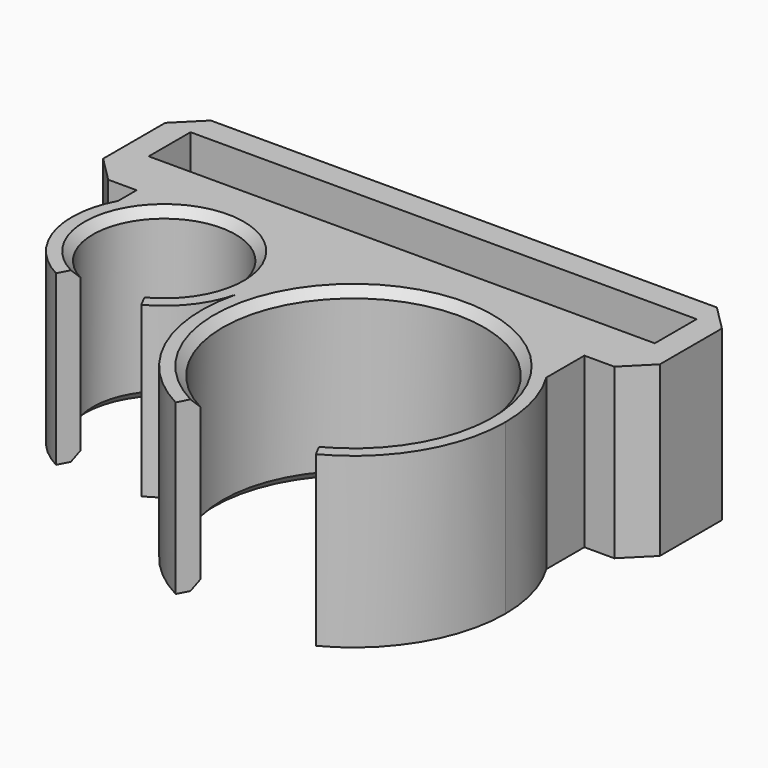
from build123d import *

# Parameters (mm, degrees)
F0_W          = 60
F0_H          = 6.2
F0_R          = 8.45
F0_R_2        = 15.5
F1_DEPTH      = 20
F2_SIZE       = 1
F4_W          = 48.1594242923
F4_H          = 40.4543727636
F5_ANGLE_BACK = 27.5
F5_ANGLE      = 55
F7_W          = 69.6530229799
F7_H          = 48.1908544898
F8_ANGLE_BACK = 27.5
F8_ANGLE      = 55
F9_SIZE       = 3
F10_SIZE      = 3
F11_SIZE      = 3
F12_SIZE      = 1
F13_TEXT_SIZE = 11.0604027416
F14_DEPTH     = 4
F15_DEPTH     = 0.8157047022


# Not quite as in the source:
# - Text() gives the source's letters only with a copy of the font that has no kerning and outlines rounded to 1/6400 em; it was checked with that copy


with BuildPart() as f1:
    # F0 (on Top) → F1 (new body)
    with BuildSketch(Plane.XY):
        Polygon((-2.1916090953, 0.4419453137), (-2.1916090953, -11.7580546863), (13.8083908874, -11.7580546863), (41.886852401, -11.7580546863), (63.8083909047, -11.7580546863), (63.8083909047, 0.4419453137), align=None)
        with Locations((30.8083909047, -5.6580546863)):
            Rectangle(F0_W, F0_H, mode=Mode.SUBTRACT)
        with BuildLine():
            ThreePointArc((24.7583909047, -22.7080546863), (21.5512101526, -14.9652354262), (13.8083908874, -11.7580546863))
            ThreePointArc((13.8083908874, -11.7580546863), (9.7556140708, -12.5356655896), (6.2784506659, -14.7580546863))
            ThreePointArc((6.2784506659, -14.7580546863), (5.1205019911, -16.0429900785), (4.1793405429, -17.4942375501))
            ThreePointArc((4.1793405429, -17.4942375501), (9.8371397339, -32.9125470372), (24.4287415748, -25.3746352015))
            ThreePointArc((24.4287415748, -25.3746352015), (24.6756660884, -24.0514943318), (24.7583909047, -22.7080546863))
        make_face()
        with Locations((13.8083909047, -22.7080546863)):
            Circle(F0_R, mode=Mode.SUBTRACT)
        with BuildLine():
            ThreePointArc((51.836726772, -14.7580546863), (47.0830048237, -12.5243667467), (41.886852401, -11.7580546863))
            ThreePointArc((41.886852401, -11.7580546863), (30.8166570713, -15.5647190895), (24.4287415748, -25.3746352015))
            ThreePointArc((24.4287415748, -25.3746352015), (39.6784587395, -47.6220687211), (59.886852401, -29.7580546863))
            ThreePointArc((59.886852401, -29.7580546863), (59.217712646, -24.8958244194), (57.26004316, -20.395095438))
            ThreePointArc((57.26004316, -20.395095438), (54.8583004314, -17.2784098198), (51.836726772, -14.7580546863))
        make_face()
        with Locations((41.886852401, -29.7580546863)):
            Circle(F0_R_2, mode=Mode.SUBTRACT)
        with BuildLine():
            Line((63.8083909047, -11.7580546863), (41.886852401, -11.7580546863))
            ThreePointArc((41.886852401, -11.7580546863), (47.0830048237, -12.5243667467), (51.836726772, -14.7580546863))
            Line((51.836726772, -14.7580546863), (57.26004316, -14.7580546863))
            Line((57.26004316, -14.7580546863), (63.8083909047, -14.7580546863))
            Line((63.8083909047, -14.7580546863), (63.8083909047, -11.7580546863))
        make_face()
        with BuildLine():
            Line((13.8083908874, -11.7580546863), (-2.1916090953, -11.7580546863))
            Line((-2.1916090953, -11.7580546863), (-2.1916090953, -14.7580546863))
            Line((-2.1916090953, -14.7580546863), (4.1793405429, -14.7580546863))
            Line((4.1793405429, -14.7580546863), (6.2784506659, -14.7580546863))
            ThreePointArc((6.2784506659, -14.7580546863), (9.7556140708, -12.5356655896), (13.8083908874, -11.7580546863))
        make_face()
        with BuildLine():
            Line((41.886852401, -11.7580546863), (13.8083908874, -11.7580546863))
            ThreePointArc((13.8083908874, -11.7580546863), (21.5512101526, -14.9652354262), (24.7583909047, -22.7080546863))
            ThreePointArc((24.7583909047, -22.7080546863), (24.6756660884, -24.0514943318), (24.4287415748, -25.3746352015))
            ThreePointArc((24.4287415748, -25.3746352015), (30.8166570713, -15.5647190895), (41.886852401, -11.7580546863))
        make_face()
        with BuildLine():
            Line((57.26004316, -14.7580546863), (51.836726772, -14.7580546863))
            ThreePointArc((51.836726772, -14.7580546863), (54.8583004314, -17.2784098198), (57.26004316, -20.395095438))
            Line((57.26004316, -20.395095438), (57.26004316, -14.7580546863))
        make_face()
        with BuildLine():
            ThreePointArc((4.1793405429, -17.4942375501), (5.1205019911, -16.0429900785), (6.2784506659, -14.7580546863))
            Line((6.2784506659, -14.7580546863), (4.1793405429, -14.7580546863))
            Line((4.1793405429, -14.7580546863), (4.1793405429, -17.4942375501))
        make_face()
    extrude(amount=F1_DEPTH)

    # F2
    f2_edges = [f1.edges().sort_by_distance(p)[0] for p in [
        (26.386852, -29.758055, 20),
        (5.358391, -22.708055, 20),
    ]]
    chamfer(f2_edges, length=F2_SIZE)

    # F4 (on plane+point) → F5 (revolve, cut)
    with BuildSketch(Plane.YZ.offset(41.886852401), mode=Mode.PRIVATE) as f5_sk:
        with Locations((-53.8377668325, 20.2271863818)):
            Rectangle(F4_W, F4_H)
    revolve(f5_sk.sketch.rotate(Axis((41.886852401, -29.7580546863, 20.2271863818), (0, 0, -1)), -F5_ANGLE_BACK), axis=Axis((41.886852401, -29.7580546863, 20.2271863818), (0, 0, -1)), revolution_arc=F5_ANGLE, mode=Mode.SUBTRACT)

    # F7 (on plane+point) → F8 (revolve, cut)
    with BuildSketch(Plane.YZ.offset(13.8083909047), mode=Mode.PRIVATE) as f8_sk:
        with Locations((-57.5345661763, 24.0954272449)):
            Rectangle(F7_W, F7_H)
    revolve(f8_sk.sketch.rotate(Axis((13.8083909047, -22.7080546863, 24.0954272449), (0, 0, -1)), -F8_ANGLE_BACK), axis=Axis((13.8083909047, -22.7080546863, 24.0954272449), (0, 0, -1)), revolution_arc=F8_ANGLE, mode=Mode.SUBTRACT)

    # F9
    f9_edges = [f1.edges().sort_by_distance(p)[0] for p in [
        (63.808391, -14.758055, 10),
    ]]
    chamfer(f9_edges, length=F9_SIZE)

    # F10
    f10_edges = [f1.edges().sort_by_distance(p)[0] for p in [
        (-2.191609, -14.758055, 10),
    ]]
    chamfer(f10_edges, length=F10_SIZE)

    # F11
    f11_edges = [f1.edges().sort_by_distance(p)[0] for p in [
        (-2.191609, 0.441945, 10),
        (63.808391, 0.441945, 10),
    ]]
    chamfer(f11_edges, length=F11_SIZE)

    # F12
    f12_edges = [f1.edges().sort_by_distance(p)[0] for p in [
        (41.886852, -14.258055, 0),
        (13.808391, -14.258055, 0),
    ]]
    chamfer(f12_edges, length=F12_SIZE)

    # F13 (on face) → F14 (cut)
    with BuildSketch(Plane(origin=(0, 0.4419453137, 0), x_dir=(-1, 0, 0), z_dir=(0, 1, 0))):
        with Locations((-41.7356863618, 5.6098985951)):
            Text('V4.1', F13_TEXT_SIZE, font='Open Sans', text_align=(TextAlign.LEFT, TextAlign.BOTTOM))
    extrude(amount=-F14_DEPTH, mode=Mode.SUBTRACT)


with BuildPart() as f15:
    # F15 (new, through all): a face of the model
    f15_faces = [f1.part.faces().sort_by_distance(p)[0] for p in [
        (32.5529598044, -1.0580546863, 8.2402006221),
    ]]
    extrude(f15_faces, amount=F15_DEPTH)


solid = Compound([f1.part, f15.part])
